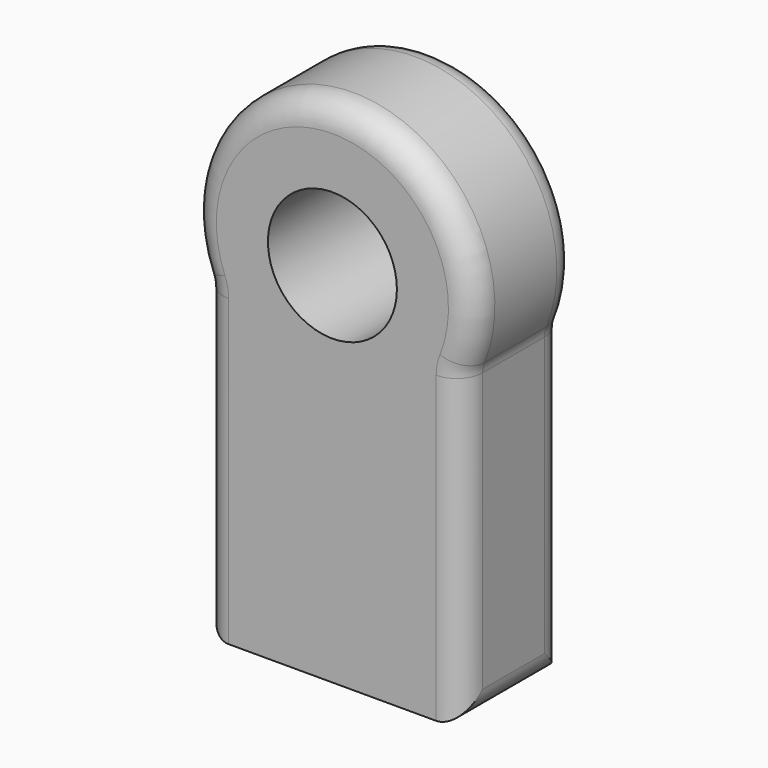
from build123d import *

# Parameters (mm, degrees)
F0_R     = 12.5
F1_DEPTH = 25
F2_R     = 5


with BuildPart() as f1:
    # F0 (on Front) → F1 (new body)
    with BuildSketch(Plane.XZ):
        with BuildLine():
            ThreePointArc((25.1206115917, 18.3788214192), (0, 57.0683197663), (-25.1206115917, 18.3788214192))
            Line((-25.1206115917, 18.3788214192), (-25.1206115917, -41.6211785808))
            Line((-25.1206115917, -41.6211785808), (25.1206115917, -41.6211785808))
            Line((25.1206115917, -41.6211785808), (25.1206115917, 18.3788214192))
        make_face()
        with Locations((0, 29.5683197663)):
            Circle(F0_R, mode=Mode.SUBTRACT)
    extrude(amount=F1_DEPTH)

    # F2
    f2_edges = [f1.edges().sort_by_distance(p)[0] for p in [
        (-25.120612, -12.5, -41.621179),
        (25.120612, -12.5, -41.621179),
        (-25.120612, -12.5, 18.378821),
        (25.120612, -12.5, 18.378821),
        (0, 0, 57.06832),
        (0, -25, 57.06832),
        (25.120612, 0, -11.621179),
        (25.120612, -25, -11.621179),
        (-25.120612, 0, -11.621179),
        (-25.120612, -25, -11.621179),
    ]]
    fillet(f2_edges, radius=F2_R)


solid = f1.part
